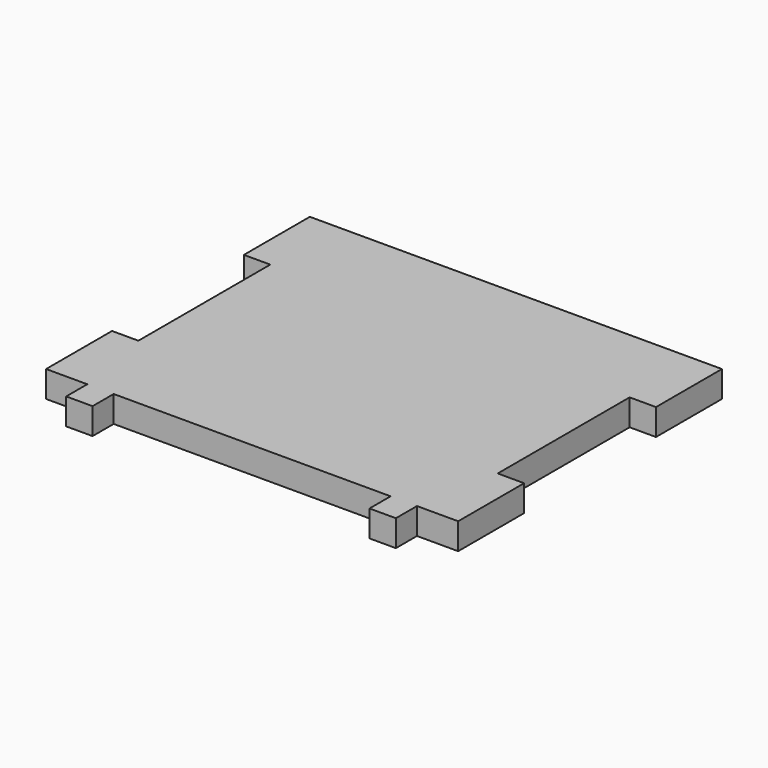
from build123d import *

# Parameters (mm, degrees)
F1_DEPTH = 4.064
F0_W     = 4.064
F0_H     = 4.064
F2_DEPTH = 4.064


# Not quite as in the source:
# - a feature names something its author has since deleted; it is built from what else it names


with BuildPart() as f1:
    # F0 (on Top) → F1 (new body)
    with BuildSketch(Plane.XY):
        Polygon((31.75, 12.7), (31.75, 25.4), (-31.75, 25.4), (-31.75, 12.7), (-27.686, 12.7), (-27.686, -12.7), (-31.75, -12.7), (-31.75, -25.4), (-25.4, -25.4), (-25.4, -21.336), (25.4, -21.336), (25.4, -25.4), (31.75, -25.4), (31.75, -12.7), (27.686, -12.7), (27.686, 12.7), align=None)
    extrude(amount=F1_DEPTH)

    # F0 (on Top) → F2 (join)
    with BuildSketch(Plane.XY):
        Polygon((21.336, -25.4), (25.4, -25.4), (25.4, -21.336), (-25.4, -21.336), (-25.4, -25.4), (-21.336, -25.4), align=None)
        with Locations((23.368, -27.432)):
            Rectangle(F0_W, F0_H)
        with Locations((-23.368, -27.432)):
            Rectangle(F0_W, F0_H)
        Polygon((31.75, 12.7), (31.75, 25.4), (-31.75, 25.4), (-31.75, 12.7), (-27.686, 12.7), (-27.686, -12.7), (-31.75, -12.7), (-31.75, -25.4), (-25.4, -25.4), (-25.4, -21.336), (25.4, -21.336), (25.4, -25.4), (31.75, -25.4), (31.75, -12.7), (27.686, -12.7), (27.686, 12.7), align=None)
    extrude(amount=F2_DEPTH)


solid = f1.part
